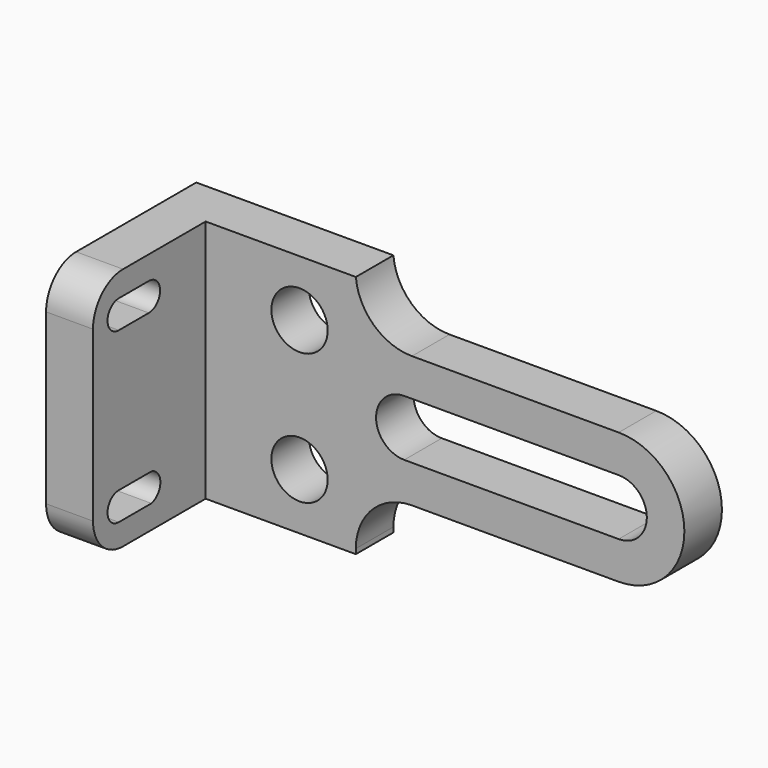
from build123d import *

# Parameters (mm, degrees)
F0_R        = 6
F1_DEPTH    = 10
F2_T1_DEPTH = 10
F3_W        = 40
F3_H        = 52
F4_DEPTH    = 10
F5_R        = 8


# Not quite as in the source:
# - a fillet or chamfer that OpenCascade refuses, or shapes differently, is made with other operations: its cross-section is extruded or revolved along the edge and cut away or added


with BuildPart() as f1:
    # F0 (on Front) → F1 (new body)
    with BuildSketch(Plane.XZ):
        with BuildLine():
            Line((32, 52), (0, 52))
            Line((0, 52), (0, 0))
            Line((0, 0), (32, 0))
            Line((32, 0), (32, 13.0432075486))
            Line((32, 13.0432075486), (88, 13.0432075486))
            ThreePointArc((88, 13.0432075486), (102, 27.0432075486), (88, 41.0432075486))
            Line((88, 41.0432075486), (32, 41.0432075486))
            Line((32, 41.0432075486), (32, 52))
        make_face()
        with Locations((20, 12)):
            Circle(F0_R, mode=Mode.SUBTRACT)
        with Locations((20, 40)):
            Circle(F0_R, mode=Mode.SUBTRACT)
        with BuildLine():
            ThreePointArc((88, 33.0432075486), (94, 27.0432075486), (88, 21.0432075486))
            Line((88, 21.0432075486), (42.3112809658, 21.0432075486))
            ThreePointArc((42.3112809658, 21.0432075486), (36.3112809658, 27.0432075486), (42.3112809658, 33.0432075486))
            Line((42.3112809658, 33.0432075486), (88, 33.0432075486))
        make_face(mode=Mode.SUBTRACT)
    extrude(amount=F1_DEPTH)

    # F2: fillet of radius 12 on 2 edges, made by hand

    # F2_s2 → F2_t1 (join)
    with BuildSketch(Plane.XZ):
        with BuildLine():
            ThreePointArc((43.9545689178, 41.0432075486), (35.8465016568, 44.1967819828), (32, 52))
            Line((32, 52), (32, 41.0432075486))
            Line((32, 41.0432075486), (43.9545689178, 41.0432075486))
        make_face()
        with BuildLine():
            ThreePointArc((32, 1.0432075486), (35.5147186258, 9.5284889228), (44, 13.0432075486))
            Line((44, 13.0432075486), (32, 13.0432075486))
            Line((32, 13.0432075486), (32, 1.0432075486))
        make_face()
    extrude(amount=F2_T1_DEPTH)

    # F3 (on face) → F4 (join)
    with BuildSketch(Plane(origin=(0, 0, 0), x_dir=(0, -1, 0), z_dir=(-1, 0, 0))):
        with Locations((20, 26)):
            Rectangle(F3_W, F3_H)
        with BuildLine():
            ThreePointArc((33.1354735655, 11), (36.1354735655, 8), (33.1354735655, 5))
            Line((33.1354735655, 5), (24.4329432571, 5))
            ThreePointArc((24.4329432571, 5), (22.054313259, 8), (24.4329432571, 11))
            Line((24.4329432571, 11), (33.1354735655, 11))
        make_face(mode=Mode.SUBTRACT)
        with BuildLine():
            ThreePointArc((33.1354735655, 47), (36.1354735655, 44), (33.1354735655, 41))
            Line((33.1354735655, 41), (25.1354735655, 41))
            ThreePointArc((25.1354735655, 41), (22.1354735655, 44), (25.1354735655, 47))
            Line((25.1354735655, 47), (33.1354735655, 47))
        make_face(mode=Mode.SUBTRACT)
    extrude(amount=F4_DEPTH)

    # F5
    f5_edges = [f1.edges().sort_by_distance(p)[0] for p in [
        (-5, -40, 52),
        (-5, -40, 0),
    ]]
    fillet(f5_edges, radius=F5_R)


solid = f1.part
